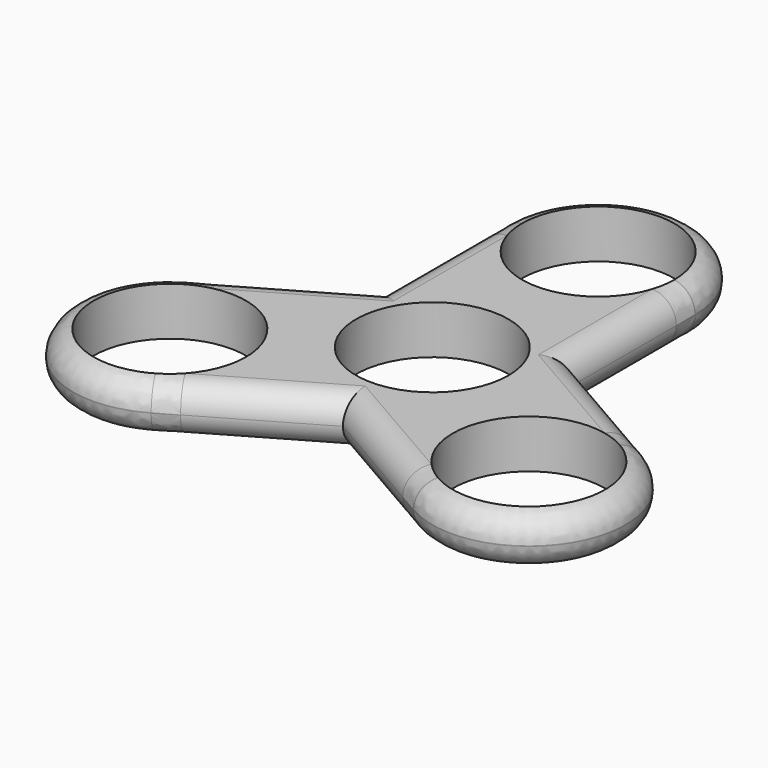
from build123d import *

# Parameters (mm, degrees)
F0_R            = 11.025
F1_DEPTH        = 7
F1_COPIES_COUNT = 3
F2_R            = 3.49999


# Not quite as in the source:
# - two fillets or chamfers of one size are made in one step
# - a fillet or chamfer is up to 0.001 mm smaller than in the source, because OpenCascade refuses the exact size
# - a feature of the source that left no trace in its solid (it failed there, or was rolled back) is left out
# - a pattern or mirror of a feature is missing from the dataset's text; its kind, count and spacing are read off the source's solid


with BuildPart() as f1:
    # F0 (on Top) → F1 (new body)
    with BuildSketch(Plane.XY):
        with BuildLine():
            Line((14, -19.4926969707), (14, 10.5073030293))
            ThreePointArc((14, 10.5073030293), (0, 24.5073030293), (-14, 10.5073030293))
            Line((-14, 10.5073030293), (-14, -19.4926969707))
            ThreePointArc((-14, -19.4926969707), (0, -33.4926969707), (14, -19.4926969707))
        make_face()
        with Locations((0, -19.4926969707)):
            Circle(F0_R, mode=Mode.SUBTRACT)
        with Locations((0, 10.5073030293)):
            Circle(F0_R, mode=Mode.SUBTRACT)
    extrude(amount=F1_DEPTH)

    # F1_copies: F1 ×3 about axis
    f1_copies_axis = Axis((0, -19.492697, 0), (0, 0, 1))


with BuildPart() as f1_1:
    add(f1.part)
    for i in range(1, F1_COPIES_COUNT):
        add(f1.part.rotate(f1_copies_axis, i * 360 / F1_COPIES_COUNT))

    # F2 (radius 3.5 in the source; OpenCascade refuses exactly that, so slightly less here)
    f2_edges = [f1_1.edges().sort_by_distance(p)[0] for p in [
        (14, -0.451245, 7),
        (-14, -0.451245, 7),
        (0, 24.507303, 7),
        (-9.490381, -41.137779, 7),
        (9.490381, -41.137779, 7),
        (23.490381, -16.889067, 7),
        (-23.490381, -16.889067, 7),
        (-23.490381, -16.889067, 0),
        (23.490381, -16.889067, 0),
        (9.490381, -41.137779, 0),
        (-9.490381, -41.137779, 0),
        (14, -0.451245, 0),
        (-14, -0.451245, 0),
    ]]
    fillet(f2_edges, radius=F2_R)


solid = f1_1.part
